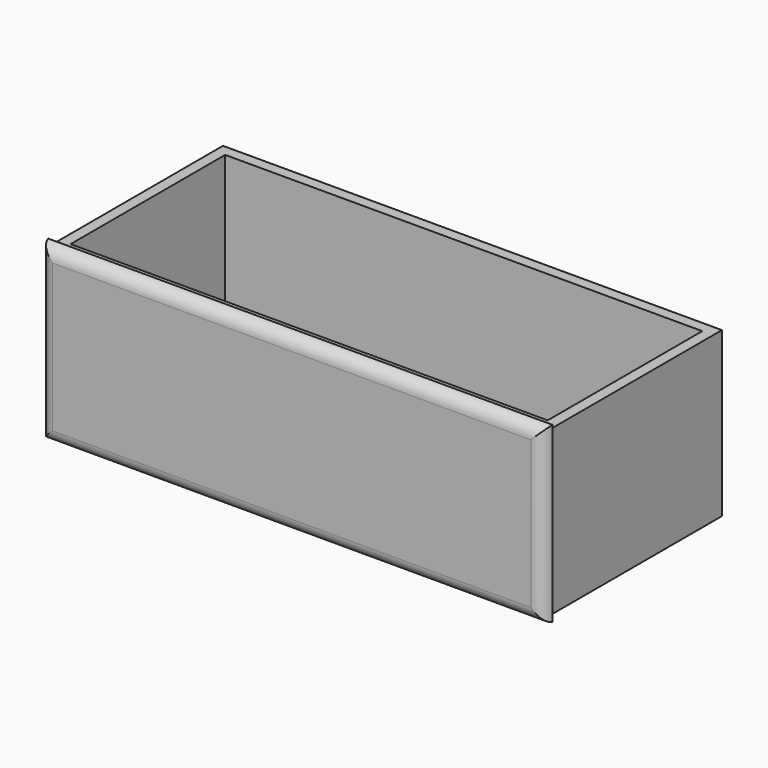
from build123d import *

# Parameters (mm, degrees)
F0_W        = 580.39
F0_H        = 250.19
F1_DEPTH    = 95.25
F2_T        = -12.7
F3_W        = 542.29
F3_H        = 171.45
F4_DEPTH    = 25.4
F5_W        = 586.74
F5_H        = 201.93
F6_DEPTH    = 12.7
F7_T1_DEPTH = 661.8742132454
F7_T3_DEPTH = 277.0642132454
F8_DEPTH    = 171.45


# Not quite as in the source:
# - a fillet or chamfer that OpenCascade refuses, or shapes differently, is made with other operations: its cross-section is extruded or revolved along the edge and cut away or added


with BuildPart() as f1:
    # F0 (on Top) → F1 (new body, symmetric)
    with BuildSketch(Plane.XY):
        Rectangle(F0_W, F0_H)
    extrude(amount=F1_DEPTH, both=True)

    # F2
    f2_openings = [f1.faces().sort_by_distance(p)[0] for p in [
        (0, 0, 95.25),
    ]]
    offset(amount=F2_T, openings=f2_openings)

    # F3 (on face) → F4 (cut)
    with BuildSketch(Plane.XZ.offset(125.095)):
        with Locations((0, 9.525)):
            Rectangle(F3_W, F3_H)
    extrude(amount=-F4_DEPTH, mode=Mode.SUBTRACT)

    # F5 (on face) → F6 (join)
    with BuildSketch(Plane.XZ.offset(125.095)):
        Rectangle(F5_W, F5_H)
        Polygon((-290.195, -95.25), (-290.195, 95.25), (-271.145, 95.25), (-271.145, -76.2), (271.145, -76.2), (271.145, 95.25), (290.195, 95.25), (290.195, -95.25), align=None, mode=Mode.SUBTRACT)
        Polygon((-271.145, 95.25), (-290.195, 95.25), (-290.195, -95.25), (290.195, -95.25), (290.195, 95.25), (271.145, 95.25), (271.145, -76.2), (-271.145, -76.2), align=None)
    extrude(amount=F6_DEPTH)

    # F7: fillet of radius 15.24 on 4 edges, made by hand

    # F7_s2 → F7_t1 (cut)
    with BuildSketch(Plane.YZ.offset(-330.9371066227)):
        with BuildLine():
            ThreePointArc((-125.095, 100.965), (-134.1947422652, 95.7755350503), (-137.795, 85.9381573509))
            Line((-137.795, 85.9381573509), (-137.795, 100.965))
            Line((-137.795, 100.965), (-125.095, 100.965))
        make_face()
        with BuildLine():
            ThreePointArc((-125.095, -100.965), (-134.1947422652, -95.7755350503), (-137.795, -85.9381573509))
            Line((-137.795, -85.9381573509), (-137.795, -100.965))
            Line((-137.795, -100.965), (-125.095, -100.965))
        make_face()
    extrude(amount=F7_T1_DEPTH, mode=Mode.SUBTRACT)

    # F7_s4 → F7_t3 (cut)
    with BuildSketch(Plane.XY.offset(-138.5321066227)):
        with BuildLine():
            ThreePointArc((-278.3431573509, -137.795), (-288.1805350503, -134.1947422652), (-293.37, -125.095))
            Line((-293.37, -125.095), (-293.37, -137.795))
            Line((-293.37, -137.795), (-278.3431573509, -137.795))
        make_face()
        with BuildLine():
            ThreePointArc((293.37, -125.095), (288.1805350503, -134.1947422652), (278.3431573509, -137.795))
            Line((278.3431573509, -137.795), (293.37, -137.795))
            Line((293.37, -137.795), (293.37, -125.095))
        make_face()
    extrude(amount=F7_T3_DEPTH, mode=Mode.SUBTRACT)

    # F8 (add): a face of the model
    f8_faces = [f1.faces().sort_by_distance(p)[0] for p in [
        (0, -118.745, -76.2),
    ]]
    extrude(f8_faces, amount=F8_DEPTH)


solid = f1.part
